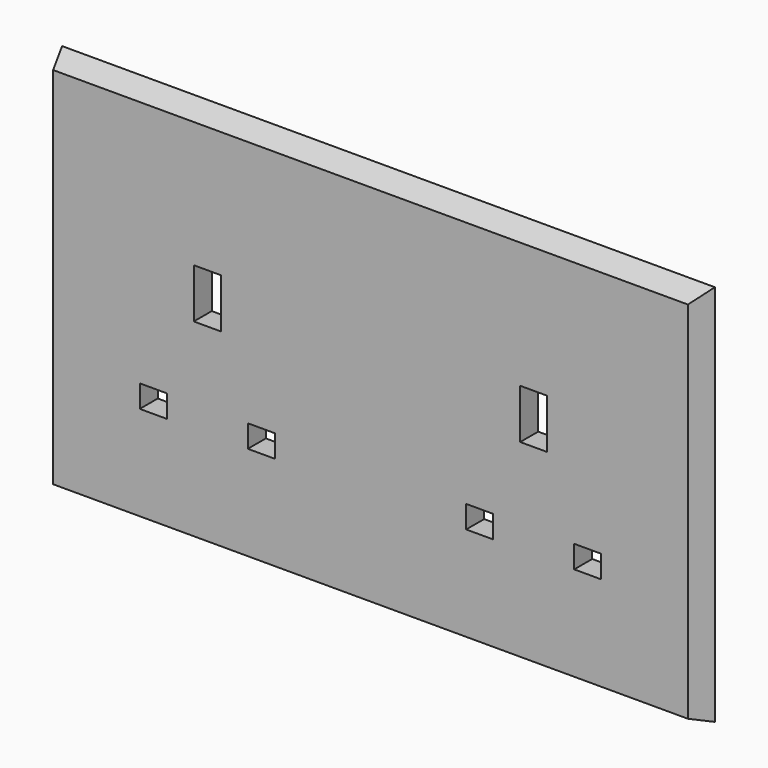
from build123d import *

# Parameters (mm, degrees)
F0_W     = 145
F0_H     = 85
F1_DEPTH = 5
F2_W     = 6
F2_H     = 11
F2_H_2   = 5
F3_DEPTH = 5
F4_SIZE2 = 4.99999
F4_SIZE  = 1.99999


# Not quite as in the source:
# - a fillet or chamfer is up to 0.001 mm smaller than in the source, because OpenCascade refuses the exact size


with BuildPart() as f1:
    # F0 (on Front) → F1 (new body)
    with BuildSketch(Plane.XZ):
        Rectangle(F0_W, F0_H)
    extrude(amount=F1_DEPTH)

    # F2 (on Front) → F3 (cut, through all)
    with BuildSketch(Plane.XZ):
        with Locations((-36.25, 7)):
            Rectangle(F2_W, F2_H)
        with Locations((-48.25, -17)):
            Rectangle(F2_W, F2_H_2)
        with Locations((-24.25, -17)):
            Rectangle(F2_W, F2_H_2)
        with Locations((36.25, 7)):
            Rectangle(F2_W, F2_H)
        with Locations((48.25, -17)):
            Rectangle(F2_W, F2_H_2)
        with Locations((24.25, -17)):
            Rectangle(F2_W, F2_H_2)
    extrude(amount=F3_DEPTH, mode=Mode.SUBTRACT)

    # F4 (size 2 and 5 in the source; OpenCascade refuses exactly that, so slightly less here)
    f4_edges = [f1.edges().sort_by_distance(p)[0] for p in [
        (0, -5, 42.5),
        (-72.5, -5, 0),
        (0, -5, -42.5),
        (72.5, -5, 0),
    ]]
    f4_side = f1.faces().sort_by_distance((0, -5, 0.092438))[0]
    chamfer(f4_edges, length=F4_SIZE, length2=F4_SIZE2, reference=f4_side)


solid = f1.part
